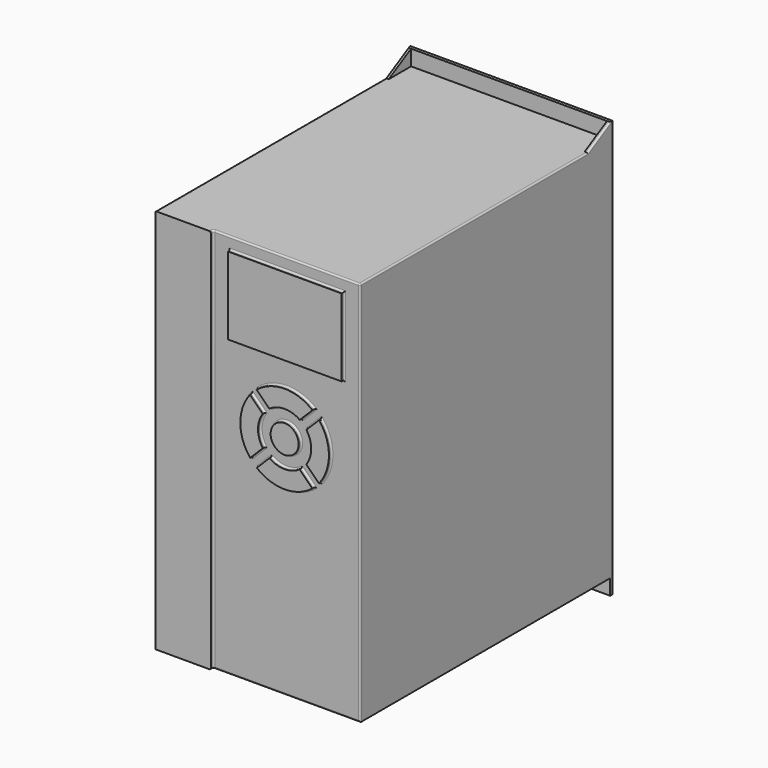
from build123d import *

# Parameters (mm, degrees)
F0_W      = 130
F0_H      = 248
F1_DEPTH  = 205
F2_W      = 94.3407235295
F2_H      = 248
F2_R      = 9
F2_W_2    = 73.0899348855
F2_H_2    = 49.802608788
F3_DEPTH  = 2
F4_W      = 130
F4_H      = 10
F5_DEPTH  = 20
F7_DEPTH  = 10
F9_DEPTH  = 130.001
F10_F1_R  = 1
F10_F2_R  = 1
F11_DEPTH = 18


with BuildPart() as f1:
    # F0 (on Front) → F1 (new body)
    with BuildSketch(Plane.XZ):
        Rectangle(F0_W, F0_H)
    extrude(amount=F1_DEPTH)

    # F2 (on face) → F3 (cut)
    with BuildSketch(Plane.XZ.offset(205)):
        with Locations((17.8296382353, 0)):
            Rectangle(F2_W, F2_H)
        with BuildLine():
            ThreePointArc((-4.041418053, 4.0888261301), (-10.3760691988, 21.9367014989), (-4.1207936375, 39.8125507927))
            Line((-4.1207936375, 39.8125507927), (4.0327052851, 31.6590518702))
            ThreePointArc((4.0327052851, 31.6590518702), (1.0381912146, 21.9360306033), (4.1054760852, 12.2357202683))
            Line((4.1054760852, 12.2357202683), (-4.041418053, 4.0888261301))
        make_face(mode=Mode.SUBTRACT)
        with BuildLine():
            Line((27.7718433373, 7.9199138179), (35.9253422598, -0.2335851046))
            ThreePointArc((35.9253422598, -0.2335851046), (18.0492121242, -6.4888600406), (0.2011808104, -0.1538563808))
            Line((0.2011808104, -0.1538563808), (8.3480462814, 7.9930090903))
            ThreePointArc((8.3480462814, 7.9930090903), (18.0485383783, 4.9254008127), (27.7718433373, 7.9199138179))
        make_face(mode=Mode.SUBTRACT)
        with Locations((18.1127931993, 22.0000017322)):
            Circle(F2_R, mode=Mode.SUBTRACT)
        with BuildLine():
            ThreePointArc((0.1029558919, 44.0740826376), (18.0492420298, 50.4888635717), (36.0239688015, 44.1542129845))
            Line((36.0239688015, 44.1542129845), (27.8770746633, 36.0073188463))
            ThreePointArc((27.8770746633, 36.0073188463), (18.0486241947, 39.0746029744), (8.2435056862, 35.9335328433))
            Line((8.2435056862, 35.9335328433), (0.1029558919, 44.0740826376))
        make_face(mode=Mode.SUBTRACT)
        with BuildLine():
            ThreePointArc((40.2666513123, 39.9116141211), (46.6016556639, 21.9367314045), (40.1868741048, 3.9901644247))
            Line((40.1868741048, 3.9901644247), (32.0463243105, 12.130714219))
            ThreePointArc((32.0463243105, 12.130714219), (35.1873955054, 21.9361164198), (32.1197858413, 31.7647486501))
            Line((32.1197858413, 31.7647486501), (40.2666513123, 39.9116141211))
        make_face(mode=Mode.SUBTRACT)
        with Locations((18.2467956167, 91.3970731086)):
            Rectangle(F2_W_2, F2_H_2, mode=Mode.SUBTRACT)
    extrude(amount=-F3_DEPTH, mode=Mode.SUBTRACT)

    # F4 (on face) → F5 (join)
    with BuildSketch(Plane(origin=(0, 0, 0), x_dir=(-1, 0, 0), z_dir=(0, 1, 0))):
        with Locations((0, 129)):
            Rectangle(F4_W, F4_H)
        with Locations((0, -129)):
            Rectangle(F4_W, F4_H)
    extrude(amount=-F5_DEPTH)

    # F6 (on face) → F7 (cut, through all)
    with BuildSketch(Plane.XY.offset(134)):
        Polygon((63, -2), (-63, -2), (-63, -20), (63, -20), (63, -18), align=None)
    extrude(amount=-F7_DEPTH, mode=Mode.SUBTRACT)

    # F8 (on face) → F9 (cut, through all)
    with BuildSketch(Plane.YZ.offset(65)):
        Polygon((-20, 134), (-20, 124), (-2, 134), align=None)
    extrude(amount=-F9_DEPTH, mode=Mode.SUBTRACT)

    # F10: fillet of radius 1 on 29 edges, made by hand

    # F10_f1
    f10_f1_edges = [f1.edges().sort_by_distance(p)[0] for p in [
        (-29.3407235295, -203, 0),
        (-0.0440441762, -203, 35.7358013315),
        (1.0381912146, -203, 21.9360306033),
        (0.0320290161, -203, 8.1622731992),
        (-10.3760691988, -203, 21.9367014989),
        (4.2746135459, -203, 3.9195763547),
        (18.0485383783, -203, 4.9254008127),
        (31.8485927986, -203, 3.8431643567),
        (18.0492121242, -203, -6.4888600406),
        (9.1127931993, -203, 22.0000017322),
        (18.0492420298, -203, 50.4888635717),
        (31.9505217324, -203, 40.0807659154),
        (18.0486241947, -203, 39.0746029744),
        (4.173230789, -203, 40.0038077405),
        (36.1932185768, -203, 35.8381813856),
        (46.6016556639, -203, 21.9367314045),
        (36.1165992076, -203, 8.0604393219),
        (35.1873955054, -203, 21.9361164198),
        (18.2467956167, -203, 66.4957687146),
        (-18.2981718261, -203, 91.3970731086),
        (18.2467956167, -203, 116.2983775027),
        (54.7917630594, -203, 91.3970731086),
    ]]
    fillet(f10_f1_edges, radius=F10_F1_R)

    # F10_f2
    f10_f2_edges = [f1.edges().sort_by_distance(p)[0] for p in [
        (-65, -112.5, 124),
        (-65, -11, 129),
        (65, -11, 129),
        (65, -111.5, 124),
        (18.3296382353, -203, 124),
        (18.3296382353, -203, -124),
        (65, -203, 0),
        (-29.0478303106, -203.2928932188, -124),
        (-29.0478303106, -203.2928932188, 124),
    ]]
    fillet(f10_f2_edges, radius=F10_F2_R)

    # F11 (cut): a face of the model
    f11_faces = [f1.faces().sort_by_distance(p)[0] for p in [
        (0, -20, -129),
    ]]
    extrude(f11_faces, amount=-F11_DEPTH, mode=Mode.SUBTRACT)


solid = f1.part
